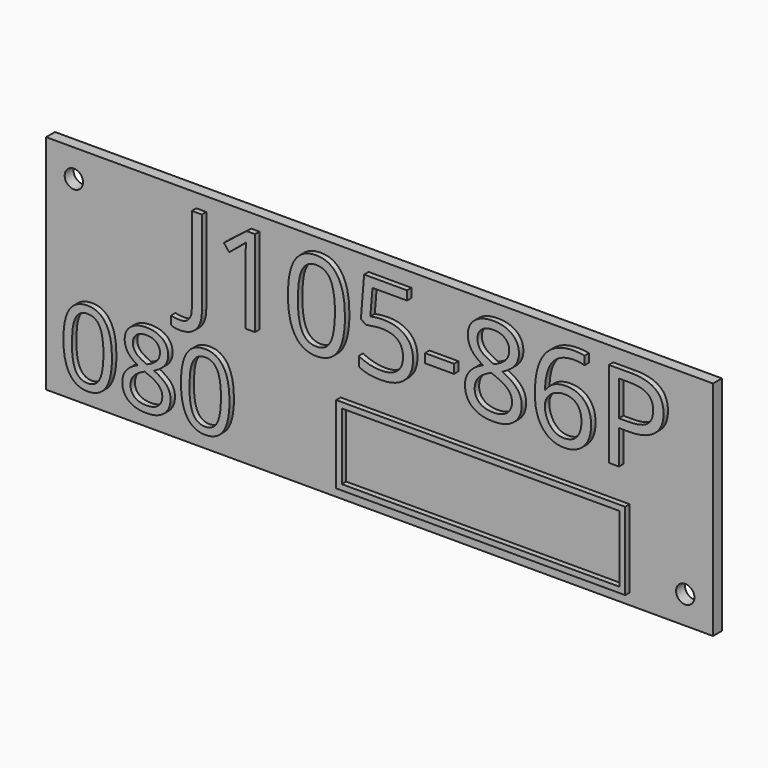
from build123d import *

# Parameters (mm, degrees)
F0_W         = 120
F0_H         = 40
F1_DEPTH     = 2
F3_D         = 3.3
F4_TEXT_SIZE = 21.733388673
F5_DEPTH     = 1
F6_TEXT_SIZE = 18.4937691891
F7_DEPTH     = 1
F8_W         = 52
F8_H         = 14
F8_W_2       = 49.99999962
F8_H_2       = 11.99999962
F9_DEPTH     = 1


# Not quite as in the source:
# - Text() gives the source's letters only with a copy of the font that has no kerning and outlines rounded to 1/6400 em; it was checked with that copy


with BuildPart() as f1:
    # F0 (on Front) → F1 (new body)
    with BuildSketch(Plane.XZ):
        Rectangle(F0_W, F0_H)
    extrude(amount=F1_DEPTH)

    # F3 (through all)
    with Locations(Plane.XZ.offset(2)):
        with Locations((-55, 15), (55, -15)):
            Hole(F3_D / 2)

    # F4 (on face) → F5 (join)
    with BuildSketch(Plane.XZ.offset(2)):
        with Locations((-35, 2)):
            Text('J105-86P', F4_TEXT_SIZE, font='Open Sans', text_align=(TextAlign.LEFT, TextAlign.BOTTOM))
    extrude(amount=F5_DEPTH)

    # F6 (on face) → F7 (join)
    with BuildSketch(Plane.XZ.offset(2)):
        with Locations((-57, -17)):
            Text('080', F6_TEXT_SIZE, font='Open Sans', text_align=(TextAlign.LEFT, TextAlign.BOTTOM))
    extrude(amount=F7_DEPTH)

    # F8 (on face) → F9 (join)
    with BuildSketch(Plane.XZ.offset(2)):
        with Locations((19, -11)):
            Rectangle(F8_W, F8_H)
        with Locations((19, -11)):
            Rectangle(F8_W_2, F8_H_2, mode=Mode.SUBTRACT)
    extrude(amount=F9_DEPTH)


solid = f1.part
